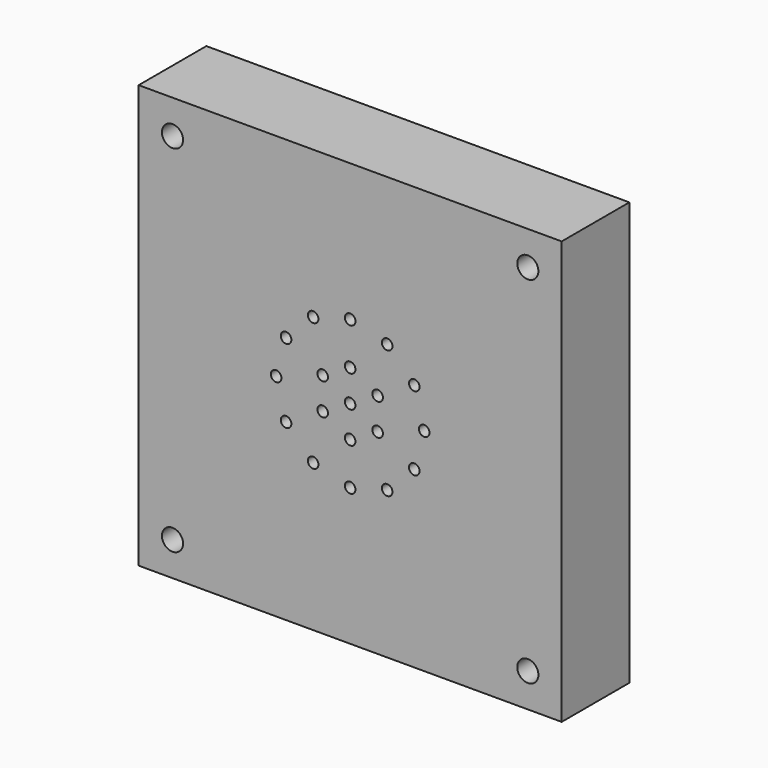
from build123d import *

# Parameters (mm, degrees)
F0_W     = 31.75
F0_H     = 31.75
F1_DEPTH = 3.175
F3_D     = 0.79375
F5_D     = 1.5875


# Not quite as in the source:
# - a feature names something its author has since deleted; it is built from what else it names


with BuildPart() as f1:
    # F0 (on Front) → F1 (new body, symmetric)
    with BuildSketch(Plane.XZ):
        Rectangle(F0_W, F0_H)
    extrude(amount=F1_DEPTH, both=True)

    # F3 (through all)
    with Locations(Plane.XZ.offset(3.175)):
        with Locations((0, 0), (0, 2.38125), (2.0622229928, 1.190625), (2.0622229928, -1.190625), (0, -2.38125), (-2.0622229928, -1.190625), (-2.0622229928, 1.190625), (-4.8118536498, 2.778125), (-2.778125, 4.8118536498), (0, 5.55625), (2.778125, 4.8118536498), (4.8118536498, 2.778125), (5.55625, 0), (4.8118536498, -2.778125), (2.778125, -4.8118536498), (0, -5.55625), (-2.778125, -4.8118536498), (-4.8118536498, -2.778125), (-5.55625, 0)):
            Hole(F3_D / 2)

    # F5 (through all)
    with Locations(Plane.XZ.offset(3.175)):
        with Locations((-13.335, 13.335), (-13.335, -13.335), (13.335, 13.335), (13.335, -13.335)):
            Hole(F5_D / 2)


solid = f1.part
